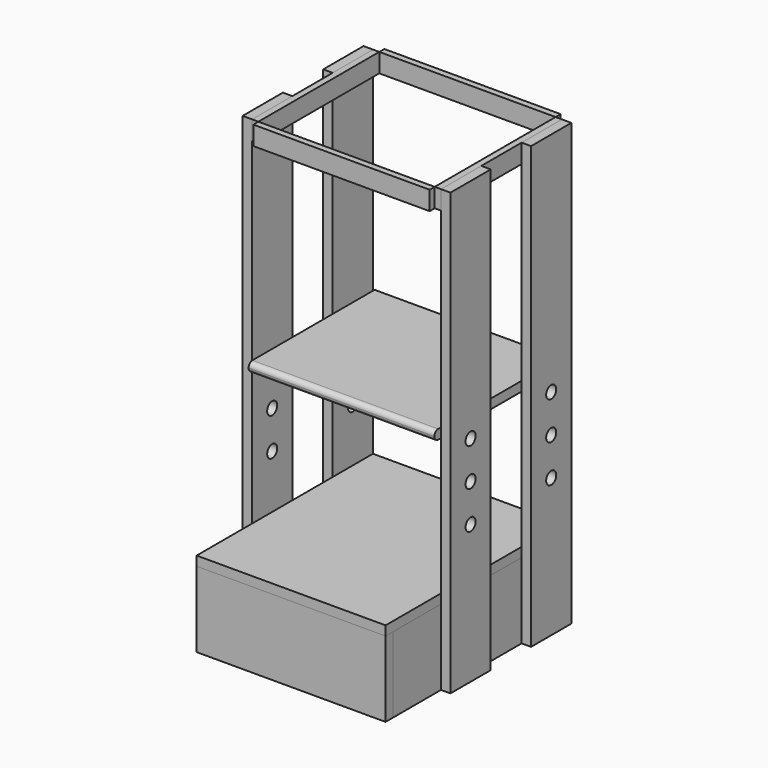
from build123d import *

# Parameters (mm, degrees)
F0_W      = 381
F0_H      = 444.5
F1_DEPTH  = 19.05
F2_W      = 381
F2_H      = 19.05
F3_DEPTH  = 152.4
F4_W      = 19.05
F4_H      = 406.4
F5_DEPTH  = 152.4
F6_W      = 101.6
F6_H      = 889
F7_DEPTH  = 19.05
F10_D     = 25.4
F10_2_D   = 25.4
F10_3_D   = 25.4
F10_4_D   = 25.4
F14_DEPTH = 19.05
F15_W     = 304.8
F15_H     = 38.1
F16_DEPTH = 12.7
F18_W     = 355.6
F18_H     = 38.1
F19_DEPTH = 12.7
F23_R     = 9.52499


# Not quite as in the source:
# - a fillet or chamfer is up to 0.001 mm smaller than in the source, because OpenCascade refuses the exact size


with BuildPart() as f1:
    # F0 (on Top) → F1 (new body)
    with BuildSketch(Plane.XY):
        Rectangle(F0_W, F0_H)
    extrude(amount=F1_DEPTH)


with BuildPart() as f3:
    # F2 (on face) → F3 (new body)
    with BuildSketch(Plane.XY):
        with Locations((0, 212.725)):
            Rectangle(F2_W, F2_H)
    extrude(amount=-F3_DEPTH)


with BuildPart() as f3b:
    # F2 (on face) → F3, piece 2 (new body)
    with BuildSketch(Plane.XY):
        with Locations((0, -212.725)):
            Rectangle(F2_W, F2_H)
    extrude(amount=-F3_DEPTH)


with BuildPart() as f5:
    # F4 (on face) → F5 (new body)
    with BuildSketch(Plane.XY):
        with Locations((-180.975, 0)):
            Rectangle(F4_W, F4_H)
    extrude(amount=-F5_DEPTH)


with BuildPart() as f5b:
    # F4 (on face) → F5, piece 2 (new body)
    with BuildSketch(Plane.XY):
        with Locations((180.975, 0)):
            Rectangle(F4_W, F4_H)
    extrude(amount=-F5_DEPTH)


with BuildPart() as f7:
    # F6 (on face) → F7 (new body)
    with BuildSketch(Plane(origin=(-190.5, 0, 0), x_dir=(0, -1, 0), z_dir=(-1, 0, 0))):
        with Locations((-171.45, 292.1)):
            Rectangle(F6_W, F6_H)
    extrude(amount=F7_DEPTH)


with BuildPart() as f7b:
    # F6 (on face) → F7, piece 2 (new body)
    with BuildSketch(Plane(origin=(-190.5, 0, 0), x_dir=(0, -1, 0), z_dir=(-1, 0, 0))):
        with Locations((31.75, 292.1)):
            Rectangle(F6_W, F6_H)
    extrude(amount=F7_DEPTH)


with BuildPart() as f8_1:
    # F8: instance of F7b
    add(f7b.part.mirror(Plane.YZ))

    # F10#3 (through all)
    with Locations(Plane(origin=(-209.55, 0, 0), x_dir=(0, -1, 0), z_dir=(-1, 0, 0))):
        with Locations((-171.45, 279.4), (31.75, 279.4), (31.75, 203.2), (-171.45, 203.2), (-171.45, 127), (31.75, 127)):
            Hole(F10_3_D / 2)


with BuildPart() as f8_2:
    # F8: instance of F7
    add(f7.part.mirror(Plane.YZ))

    # F10#4 (through all)
    with Locations(Plane(origin=(-209.55, 0, 0), x_dir=(0, -1, 0), z_dir=(-1, 0, 0))):
        with Locations((-171.45, 279.4), (31.75, 279.4), (31.75, 203.2), (-171.45, 203.2), (-171.45, 127), (31.75, 127)):
            Hole(F10_4_D / 2)


with BuildPart() as f7_1:
    add(f7.part)

    # F10 (through all)
    with Locations(Plane(origin=(-209.55, 0, 0), x_dir=(0, -1, 0), z_dir=(-1, 0, 0))):
        with Locations((-171.45, 279.4), (31.75, 279.4), (31.75, 203.2), (-171.45, 203.2), (-171.45, 127), (31.75, 127)):
            Hole(F10_D / 2)


with BuildPart() as f7b_1:
    add(f7b.part)

    # F10#2 (through all)
    with Locations(Plane(origin=(-209.55, 0, 0), x_dir=(0, -1, 0), z_dir=(-1, 0, 0))):
        with Locations((-171.45, 279.4), (31.75, 279.4), (31.75, 203.2), (-171.45, 203.2), (-171.45, 127), (31.75, 127)):
            Hole(F10_2_D / 2)


with BuildPart() as f14:
    # F13 (on plane+point) → F14 (new body)
    with BuildSketch(Plane.XY.offset(292.1)):
        Polygon((-187.325, -95.25), (187.325, -95.25), (187.325, -26.0919403405), (187.325, 222.25), (-187.325, 222.25), (-187.325, -82.55), align=None)
    extrude(amount=F14_DEPTH)

    # F23 (radius 9.525 in the source; OpenCascade refuses exactly that, so slightly less here)
    f23_edges = [f14.edges().sort_by_distance(p)[0] for p in [
        (0, -95.25, 311.15),
        (0, -95.25, 292.1),
    ]]
    fillet(f23_edges, radius=F23_R)


with BuildPart() as f16:
    # F15 (on face) → F16 (new body)
    with BuildSketch(Plane.YZ.offset(-190.5)):
        with Locations((69.85, 717.55)):
            Rectangle(F15_W, F15_H)
    extrude(amount=F16_DEPTH)


with BuildPart() as f17_1:
    # F17: instance of F16
    add(f16.part.mirror(Plane.YZ))


with BuildPart() as f19:
    # F18 (on face) → F19 (new body)
    with BuildSketch(Plane.XZ.offset(82.55)):
        with Locations((0, 717.55)):
            Rectangle(F18_W, F18_H)
    extrude(amount=F19_DEPTH)


with BuildPart() as f22_1:
    # F22: instance of F19
    add(f19.part.mirror(Plane.XZ.offset(-69.85)))


solid = Compound([f1.part, f3.part, f3b.part, f5.part, f5b.part, f8_1.part, f8_2.part, f7_1.part, f7b_1.part, f14.part, f16.part, f17_1.part, f19.part, f22_1.part])
